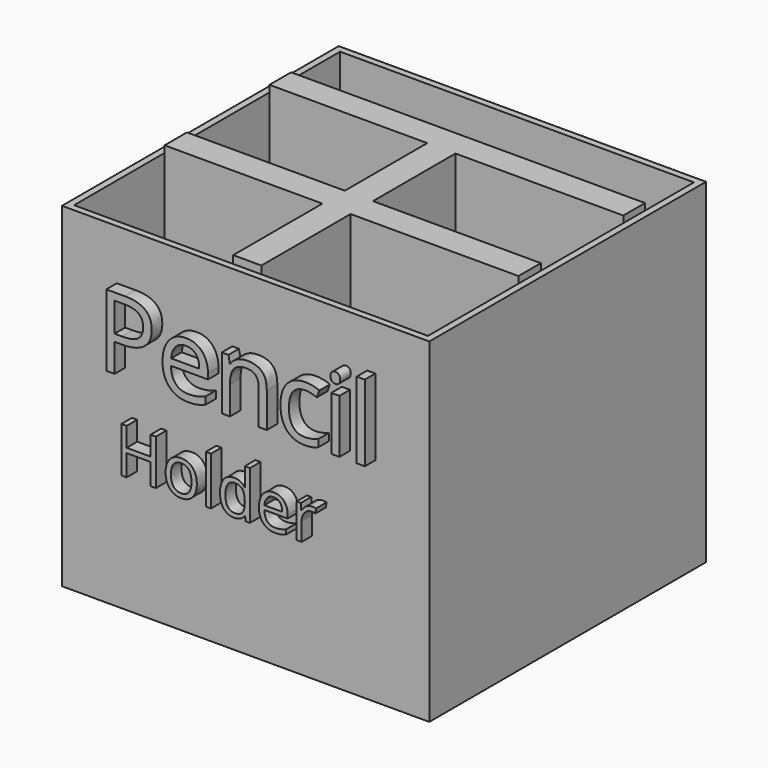
from build123d import *

# Parameters (mm, degrees)
F0_W         = 139.2736807466
F0_H         = 131.1470344663
F1_DEPTH     = 127
F2_T         = -2.54
F3_TEXT_SIZE = 38.0767302381
F4_DEPTH     = 5
F5_TEXT_SIZE = 24.0783051898
F6_DEPTH     = 5
F7_W         = 134.1936807466
F7_H         = 10.2704353631
F8_DEPTH     = 127
F9_W         = 134.1936807466
F9_H         = 10.6017384678
F10_DEPTH    = 127
F11_W        = 10.6845669216
F11_H        = 102.2479459643
F12_DEPTH    = 127


# Not quite as in the source:
# - Text() gives the source's letters only with a copy of the font that has no kerning and outlines rounded to 1/6400 em; it was checked with that copy


with BuildPart() as f1:
    # F0 (on Top) → F1 (new body)
    with BuildSketch(Plane.XY):
        with Locations((-1.5733502805, 0.4157014191)):
            Rectangle(F0_W, F0_H)
    extrude(amount=F1_DEPTH)

    # F2
    f2_openings = [f1.faces().sort_by_distance(p)[0] for p in [
        (-1.57335, 0.415701, 127),
    ]]
    offset(amount=F2_T, openings=f2_openings)

    # F3 (on face) → F4 (join)
    with BuildSketch(Plane.XZ.offset(65.157815814)):
        with Locations((-54.159399122, 80.7179361582)):
            Text('Pencil', F3_TEXT_SIZE, font='Open Sans', text_align=(TextAlign.LEFT, TextAlign.BOTTOM))
    extrude(amount=F4_DEPTH)

    # F5 (on face) → F6 (join)
    with BuildSketch(Plane.XZ.offset(65.157815814)):
        with Locations((-47.0482558012, 47.6564876735)):
            Text('Holder', F5_TEXT_SIZE, font='Open Sans', text_align=(TextAlign.LEFT, TextAlign.BOTTOM))
    extrude(amount=F6_DEPTH)

    # F7 (on face) → F8 (join)
    with BuildSketch(Plane.XY.offset(2.54)):
        with Locations((-1.5733502805, 35.1148117334)):
            Rectangle(F7_W, F7_H)
    extrude(amount=F8_DEPTH)

    # F9 (on face) → F10 (join)
    with BuildSketch(Plane.XY.offset(2.54)):
        with Locations((-1.5733502805, -14.4151886925)):
            Rectangle(F9_W, F9_H)
    extrude(amount=F10_DEPTH)

    # F11 (on face) → F12 (join)
    with BuildSketch(Plane.XY.offset(2.54)):
        with Locations((-3.4786954639, -10.8739435673)):
            Rectangle(F11_W, F11_H)
    extrude(amount=F12_DEPTH)


solid = f1.part
